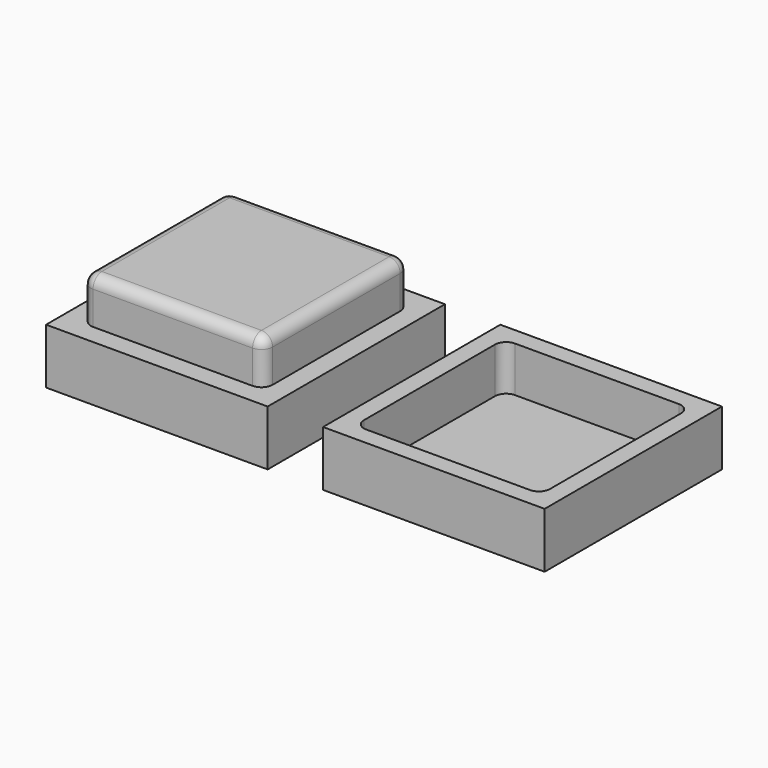
from build123d import *

# Parameters (mm, degrees)
F0_W         = 20
F0_H         = 20
F1_DEPTH     = 5
F2_W         = 16.4
F2_H         = 16.4
F3_DEPTH     = 4
F4_R         = 1
F5_W         = 20
F5_H         = 20
F6_DEPTH     = 5
F7_W         = 16.8
F7_H         = 16.8
F8_DEPTH     = 4.1
F9_T1_DEPTH  = 3
F9_S5_W      = 1
F9_S5_H      = 1
F9_T6_DEPTH  = 1
F9_S11_W     = 1
F9_S11_H     = 1
F9_T12_DEPTH = 1
F9_S17_W     = 1
F9_S17_H     = 1
F9_T18_DEPTH = 1
F9_S23_W     = 1
F9_S23_H     = 1
F9_T24_DEPTH = 1
F10_R        = 1


# Not quite as in the source:
# - a fillet or chamfer that OpenCascade refuses, or shapes differently, is made with other operations: its cross-section is extruded or revolved along the edge and cut away or added


with BuildPart() as f1:
    # F0 (on Top) → F1 (new body)
    with BuildSketch(Plane.XY):
        with Locations((-10, 10)):
            Rectangle(F0_W, F0_H)
    extrude(amount=F1_DEPTH)

    # F2 (on face) → F3 (join)
    with BuildSketch(Plane.XY.offset(5)):
        with Locations((-10, 10)):
            Rectangle(F2_W, F2_H)
    extrude(amount=F3_DEPTH)

    # F4
    f4_edges = [f1.edges().sort_by_distance(p)[0] for p in [
        (-10, 1.8, 9),
        (-1.8, 10, 9),
        (-10, 18.2, 9),
        (-18.2, 10, 9),
    ]]
    fillet(f4_edges, radius=F4_R)

    # F9: fillet of radius 1 on 4 edges, made by hand

    # F9_s2 → F9_t1 (cut)
    with BuildSketch(Plane.XY.offset(5)):
        with BuildLine():
            ThreePointArc((-1.8, 17.2), (-2.0928932188, 17.9071067812), (-2.8, 18.2))
            Line((-2.8, 18.2), (-1.8, 18.2))
            Line((-1.8, 18.2), (-1.8, 17.2))
        make_face()
        with BuildLine():
            ThreePointArc((-2.8, 1.8), (-2.0928932188, 2.0928932188), (-1.8, 2.8))
            Line((-1.8, 2.8), (-1.8, 1.8))
            Line((-1.8, 1.8), (-2.8, 1.8))
        make_face()
        with BuildLine():
            ThreePointArc((-17.2, 1.8), (-17.9071067812, 2.0928932188), (-18.2, 2.8))
            Line((-18.2, 2.8), (-18.2, 1.8))
            Line((-18.2, 1.8), (-17.2, 1.8))
        make_face()
        with BuildLine():
            ThreePointArc((-18.2, 17.2), (-17.9071067812, 17.9071067812), (-17.2, 18.2))
            Line((-17.2, 18.2), (-18.2, 18.2))
            Line((-18.2, 18.2), (-18.2, 17.2))
        make_face()
    extrude(amount=F9_T1_DEPTH, mode=Mode.SUBTRACT)


with BuildPart() as f6:
    # F5 (on Top) → F6 (new body)
    with BuildSketch(Plane.XY):
        with Locations((15, 10)):
            Rectangle(F5_W, F5_H)
    extrude(amount=F6_DEPTH)

    # F7 (on face) → F8 (cut)
    with BuildSketch(Plane.XY.offset(5)):
        with Locations((15, 10)):
            Rectangle(F7_W, F7_H)
    extrude(amount=-F8_DEPTH, mode=Mode.SUBTRACT)

    # F10
    f10_edges = [f6.edges().sort_by_distance(p)[0] for p in [
        (6.6, 18.4, 2.95),
        (23.4, 18.4, 2.95),
        (23.4, 1.6, 2.95),
        (6.6, 1.6, 2.95),
    ]]
    fillet(f10_edges, radius=F10_R)


with BuildPart() as f9_tool4:
    # F9_s5 → F9_t6 (new body)
    with BuildSketch(Plane.YZ.offset(-17.2)):
        with Locations((17.7, 8.5)):
            Rectangle(F9_S5_W, F9_S5_H)
    extrude(amount=-F9_T6_DEPTH)

    # F9_s7 → F9_t8 (revolve, cut)
    with BuildSketch(Plane(origin=(-17.2, 17.2, 8), x_dir=(0, -0.7071067812, -0.7071067812), z_dir=(0, 0.7071067812, -0.7071067812))):
        with BuildLine():
            ThreePointArc((0, -1), (1, 0), (0, 1))
            Line((0, 1), (0, -1))
        make_face()
    revolve(axis=Axis((-17.2, 17.2, 8), (-1, 0, 0)), mode=Mode.SUBTRACT)


with BuildPart() as f1_1:
    add(f1.part)

    # F9_t3: cut F9_tool4
    add(f9_tool4.part, mode=Mode.SUBTRACT)


with BuildPart() as f9_tool10:
    # F9_s11 → F9_t12 (new body)
    with BuildSketch(Plane.XZ.offset(-2.8)):
        with Locations((-17.7, 8.5)):
            Rectangle(F9_S11_W, F9_S11_H)
    extrude(amount=F9_T12_DEPTH)

    # F9_s13 → F9_t14 (revolve, cut)
    with BuildSketch(Plane(origin=(-17.2, 2.8, 8), x_dir=(0.7071067812, 0, -0.7071067812), z_dir=(-0.7071067812, 0, -0.7071067812))):
        with BuildLine():
            ThreePointArc((0, -1), (1, 0), (0, 1))
            Line((0, 1), (0, -1))
        make_face()
    revolve(axis=Axis((-17.2, 2.8, 8), (0, -1, 0)), mode=Mode.SUBTRACT)


with BuildPart() as f1_2:
    add(f1_1.part)

    # F9_t9: cut F9_tool10
    add(f9_tool10.part, mode=Mode.SUBTRACT)


with BuildPart() as f9_tool16:
    # F9_s17 → F9_t18 (new body)
    with BuildSketch(Plane.XZ.offset(-2.8)):
        with Locations((-2.3, 8.5)):
            Rectangle(F9_S17_W, F9_S17_H)
    extrude(amount=F9_T18_DEPTH)

    # F9_s19 → F9_t20 (revolve, cut)
    with BuildSketch(Plane(origin=(-2.8, 2.8, 8), x_dir=(-0.7071067812, 0, -0.7071067812), z_dir=(-0.7071067812, 0, 0.7071067812))):
        with BuildLine():
            ThreePointArc((0, -1), (1, 0), (0, 1))
            Line((0, 1), (0, -1))
        make_face()
    revolve(axis=Axis((-2.8, 2.8, 8), (0, -1, 0)), mode=Mode.SUBTRACT)


with BuildPart() as f1_3:
    add(f1_2.part)

    # F9_t15: cut F9_tool16
    add(f9_tool16.part, mode=Mode.SUBTRACT)


with BuildPart() as f9_tool22:
    # F9_s23 → F9_t24 (new body)
    with BuildSketch(Plane.YZ.offset(-2.8)):
        with Locations((17.7, 8.5)):
            Rectangle(F9_S23_W, F9_S23_H)
    extrude(amount=F9_T24_DEPTH)

    # F9_s25 → F9_t26 (revolve, cut)
    with BuildSketch(Plane(origin=(-2.8, 17.2, 8), x_dir=(0, -0.7071067812, -0.7071067812), z_dir=(0, -0.7071067812, 0.7071067812))):
        with BuildLine():
            ThreePointArc((0, -1), (1, 0), (0, 1))
            Line((0, 1), (0, -1))
        make_face()
    revolve(axis=Axis((-2.8, 17.2, 8), (1, 0, 0)), mode=Mode.SUBTRACT)


with BuildPart() as f1_4:
    add(f1_3.part)

    # F9_t21: cut F9_tool22
    add(f9_tool22.part, mode=Mode.SUBTRACT)


solid = Compound([f6.part, f1_4.part])
